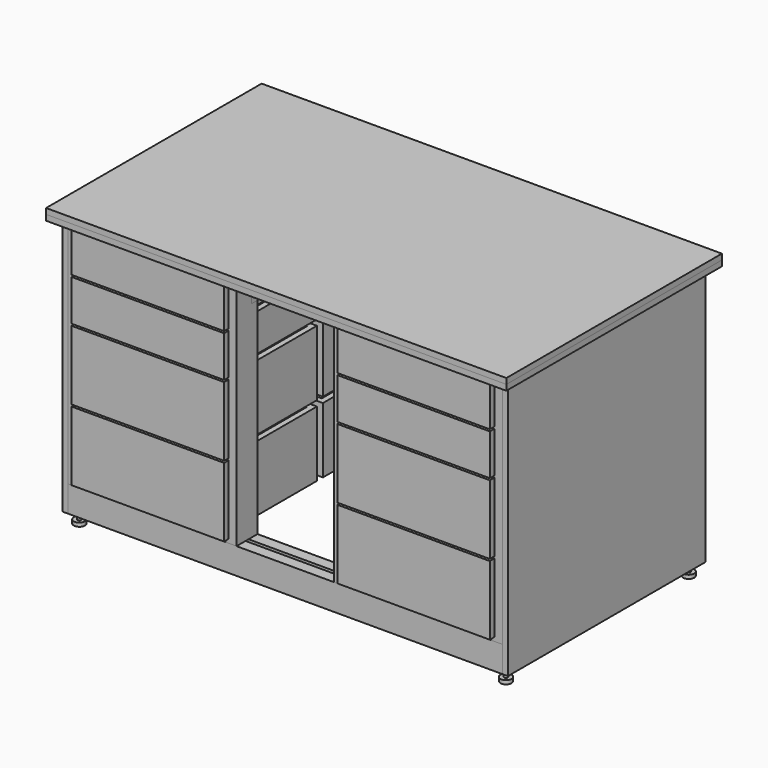
from build123d import *

# Parameters (mm, degrees)
F0_W      = 38.1
F0_H      = 88.9
F1_DEPTH  = 787.4
F2_W      = 38.1
F2_H      = 38.1
F2_W_2    = 1435.1
F3_DEPTH  = 88.9
F2_W_3    = 1473.2
F4_W      = 19.05
F4_H      = 838.2
F5_DEPTH  = 876.3
F6_W      = 38.1
F6_H      = 25.4
F7_DEPTH  = 88.9
F8_W      = 38.1
F8_H      = 685.8
F8_H_2    = 25.4
F9_DEPTH  = 88.9
F8_H_3    = 711.2
F11_DEPTH = 876.3
F12_DEPTH = 38.1
F10_W     = 1562.1
F10_H     = 19.05
F13_DEPTH = 876.3
F14_DEPTH = 38.1
F15_W     = 428.625
F15_H     = 127
F16_DEPTH = 19.05
F18_DEPTH = 127
F19_W     = 428.625
F19_H     = 368.3
F20_DEPTH = 9.525
F21_W     = 466.725
F21_H     = 127
F22_DEPTH = 19.05
F25_W     = 428.625
F25_H     = 222.25
F26_DEPTH = 19.05
F28_DEPTH = 222.25
F29_W     = 428.625
F29_H     = 368.3
F30_DEPTH = 19.05
F31_W     = 517.525
F31_H     = 234.95
F32_DEPTH = 19.05
F61_W     = 76.2
F61_H     = 12.7
F62_DEPTH = 88.9
F63_R     = 6.35
F64_DEPTH = 25.4
F65_R     = 19.05
F66_DEPTH = 12.7


# Not quite as in the source:
# - a feature names something its author has since deleted; it is built from what else it names


with BuildPart() as f1:
    # F0 (on Top) → F1 (new body)
    with BuildSketch(Plane.XY):
        with Locations((-717.55, 374.65)):
            Rectangle(F0_W, F0_H)
    extrude(amount=F1_DEPTH)


with BuildPart() as f1b:
    # F0 (on Top) → F1, piece 2 (new body)
    with BuildSketch(Plane.XY):
        with Locations((717.55, 374.65)):
            Rectangle(F0_W, F0_H)
    extrude(amount=F1_DEPTH)


with BuildPart() as f1c:
    # F0 (on Top) → F1, piece 3 (new body)
    with BuildSketch(Plane.XY):
        with Locations((717.55, -374.65)):
            Rectangle(F0_W, F0_H)
    extrude(amount=F1_DEPTH)


with BuildPart() as f1d:
    # F0 (on Top) → F1, piece 4 (new body)
    with BuildSketch(Plane.XY):
        with Locations((-717.55, -374.65)):
            Rectangle(F0_W, F0_H)
    extrude(amount=F1_DEPTH)


with BuildPart() as f1e:
    # F0 (on Top) → F1, piece 5 (new body)
    with BuildSketch(Plane.XY):
        with Locations((-184.15, 374.65)):
            Rectangle(F0_W, F0_H)
    extrude(amount=F1_DEPTH)


with BuildPart() as f1f:
    # F0 (on Top) → F1, piece 6 (new body)
    with BuildSketch(Plane.XY):
        with Locations((184.15, 374.65)):
            Rectangle(F0_W, F0_H)
    extrude(amount=F1_DEPTH)


with BuildPart() as f1g:
    # F0 (on Top) → F1, piece 7 (new body)
    with BuildSketch(Plane.XY):
        with Locations((184.15, -374.65)):
            Rectangle(F0_W, F0_H)
    extrude(amount=F1_DEPTH)


with BuildPart() as f1h:
    # F0 (on Top) → F1, piece 8 (new body)
    with BuildSketch(Plane.XY):
        with Locations((-184.15, -374.65)):
            Rectangle(F0_W, F0_H)
    extrude(amount=F1_DEPTH)


with BuildPart() as f3:
    # F2 (on face) → F3 (new body)
    with BuildSketch(Plane(origin=(0, 0, 0), x_dir=(1, 0, 0), z_dir=(0, 0, -1))):
        with Locations((-717.55, 349.25)):
            Rectangle(F2_W, F2_H)
        with Locations((19.05, 349.25)):
            Rectangle(F2_W_2, F2_H)
    extrude(amount=F3_DEPTH)


with BuildPart() as f3b:
    # F2 (on face) → F3, piece 2 (new body)
    with BuildSketch(Plane(origin=(0, 0, 0), x_dir=(1, 0, 0), z_dir=(0, 0, -1))):
        with Locations((19.05, 400.05)):
            Rectangle(F2_W_2, F2_H)
        with Locations((-717.55, 400.05)):
            Rectangle(F2_W, F2_H)
    extrude(amount=F3_DEPTH)


with BuildPart() as f3c:
    # F2 (on face) → F3, piece 3 (new body)
    with BuildSketch(Plane(origin=(0, 0, 0), x_dir=(1, 0, 0), z_dir=(0, 0, -1))):
        with Locations((0, -349.25)):
            Rectangle(F2_W_3, F2_H)
    extrude(amount=F3_DEPTH)


with BuildPart() as f3d:
    # F2 (on face) → F3, piece 4 (new body)
    with BuildSketch(Plane(origin=(0, 0, 0), x_dir=(1, 0, 0), z_dir=(0, 0, -1))):
        with Locations((0, -400.05)):
            Rectangle(F2_W_3, F2_H)
    extrude(amount=F3_DEPTH)


with BuildPart() as f5:
    # F4 (on face) → F5 (new body)
    with BuildSketch(Plane.XY.offset(787.4)):
        with Locations((746.125, 0)):
            Rectangle(F4_W, F4_H)
    extrude(amount=-F5_DEPTH)


with BuildPart() as f5b:
    # F4 (on face) → F5, piece 2 (new body)
    with BuildSketch(Plane.XY.offset(787.4)):
        Polygon((-736.6, 419.1), (-755.65, 419.1), (-755.65, -419.1), (-736.6, -419.1), (-736.6, 330.2), align=None)
    extrude(amount=-F5_DEPTH)


with BuildPart() as f7_tool:
    # F6 (on face) → F7 (new body)
    with BuildSketch(Plane.XY.offset(787.4)):
        with Locations((-717.55, 342.9)):
            Rectangle(F6_W, F6_H)
        with Locations((-184.15, 342.9)):
            Rectangle(F6_W, F6_H)
        with Locations((184.15, 342.9)):
            Rectangle(F6_W, F6_H)
        with Locations((717.55, 342.9)):
            Rectangle(F6_W, F6_H)
        with Locations((717.55, -342.9)):
            Rectangle(F6_W, F6_H)
        with Locations((184.15, -342.9)):
            Rectangle(F6_W, F6_H)
        with Locations((-184.15, -342.9)):
            Rectangle(F6_W, F6_H)
        with Locations((-717.55, -342.9)):
            Rectangle(F6_W, F6_H)
    extrude(amount=-F7_DEPTH)


with BuildPart() as f1_1:
    add(f1.part)

    # F7: cut by f7_tool
    add(f7_tool.part, mode=Mode.SUBTRACT)


with BuildPart() as f1b_1:
    add(f1b.part)

    # F7: cut by f7_tool
    add(f7_tool.part, mode=Mode.SUBTRACT)


with BuildPart() as f1c_1:
    add(f1c.part)

    # F7: cut by f7_tool
    add(f7_tool.part, mode=Mode.SUBTRACT)


with BuildPart() as f1d_1:
    add(f1d.part)

    # F7: cut by f7_tool
    add(f7_tool.part, mode=Mode.SUBTRACT)


with BuildPart() as f1e_1:
    add(f1e.part)

    # F7: cut by f7_tool
    add(f7_tool.part, mode=Mode.SUBTRACT)


with BuildPart() as f1f_1:
    add(f1f.part)

    # F7: cut by f7_tool
    add(f7_tool.part, mode=Mode.SUBTRACT)


with BuildPart() as f1g_1:
    add(f1g.part)

    # F7: cut by f7_tool
    add(f7_tool.part, mode=Mode.SUBTRACT)


with BuildPart() as f1h_1:
    add(f1h.part)

    # F7: cut by f7_tool
    add(f7_tool.part, mode=Mode.SUBTRACT)


with BuildPart() as f9:
    # F8 (on face) → F9 (new body)
    with BuildSketch(Plane.XY.offset(698.5)):
        with Locations((-717.55, -12.7)):
            Rectangle(F8_W, F8_H)
        with Locations((-717.55, 342.9)):
            Rectangle(F8_W, F8_H_2)
    extrude(amount=F9_DEPTH)


with BuildPart() as f9b:
    # F8 (on face) → F9, piece 2 (new body)
    with BuildSketch(Plane.XY.offset(698.5)):
        with Locations((-184.15, 0)):
            Rectangle(F8_W, F8_H_3)
    extrude(amount=F9_DEPTH)


with BuildPart() as f9c:
    # F8 (on face) → F9, piece 3 (new body)
    with BuildSketch(Plane.XY.offset(698.5)):
        with Locations((184.15, 0)):
            Rectangle(F8_W, F8_H_3)
    extrude(amount=F9_DEPTH)


with BuildPart() as f9d:
    # F8 (on face) → F9, piece 4 (new body)
    with BuildSketch(Plane.XY.offset(698.5)):
        with Locations((717.55, 0)):
            Rectangle(F8_W, F8_H_3)
    extrude(amount=F9_DEPTH)


with BuildPart() as f11:
    # F10 (on face) → F11 (new body)
    with BuildSketch(Plane.XZ.offset(419.1)):
        Polygon((781.05, 806.45), (-781.05, 806.45), (-781.05, 787.4), (-736.6, 787.4), (-698.5, 787.4), (781.05, 787.4), align=None)
    extrude(amount=-F11_DEPTH)

    # F10 (on face) → F12 (join)
    with BuildSketch(Plane.XZ.offset(419.1)):
        Polygon((781.05, 806.45), (-781.05, 806.45), (-781.05, 787.4), (-736.6, 787.4), (-698.5, 787.4), (781.05, 787.4), align=None)
    extrude(amount=F12_DEPTH)


with BuildPart() as f13:
    # F10 (on face) → F13 (new body)
    with BuildSketch(Plane.XZ.offset(419.1)):
        with Locations((0, 815.975)):
            Rectangle(F10_W, F10_H)
    extrude(amount=-F13_DEPTH)

    # F10 (on face) → F14 (join)
    with BuildSketch(Plane.XZ.offset(419.1)):
        with Locations((0, 815.975)):
            Rectangle(F10_W, F10_H)
    extrude(amount=F14_DEPTH)


with BuildPart() as f16:
    # F15 (on face) → F16 (new body)
    with BuildSketch(Plane.XZ.offset(419.1)):
        with Locations((-450.85, 704.85)):
            Rectangle(F15_W, F15_H)
    extrude(amount=-F16_DEPTH)

    # F17 (on face) → F18 (join)
    with BuildSketch(Plane.XY.offset(768.35)):
        Polygon((-665.1625, -400.05), (-665.1625, -31.75), (-684.2125, -31.75), (-684.2125, -419.1), (-665.1625, -419.1), align=None)
        Polygon((-217.4875, -31.75), (-236.5375, -31.75), (-236.5375, -400.05), (-236.5375, -419.1), (-217.4875, -419.1), align=None)
        Polygon((-665.1625, -31.75), (-236.5375, -31.75), (-217.4875, -31.75), (-217.4875, -12.7), (-684.2125, -12.7), (-684.2125, -31.75), align=None)
    extrude(amount=-F18_DEPTH)

    # F19 (on face) → F20 (join)
    with BuildSketch(Plane(origin=(0, 0, 641.35), x_dir=(1, 0, 0), z_dir=(0, 0, -1))):
        with Locations((-450.85, 215.9)):
            Rectangle(F19_W, F19_H)
    extrude(amount=-F20_DEPTH)


with BuildPart() as f22:
    # F21 (on face) → F22 (new body)
    with BuildSketch(Plane.XZ.offset(419.1)):
        with Locations((-450.85, 704.85)):
            Rectangle(F21_W, F21_H)
        Polygon((-192.0875, 781.05), (-709.6125, 781.05), (-709.6125, 641.35), (-684.2125, 641.35), (-684.2125, 768.35), (-217.4875, 768.35), (-217.4875, 641.35), (-192.0875, 641.35), align=None)
    extrude(amount=F22_DEPTH)


with BuildPart() as f23_1:
    # F23: copy of F16
    add(f16.part.moved(Location((0, 0, -146.05))))


with BuildPart() as f24_1:
    # F24: copy of F22
    add(f22.part.moved(Location((0, 0, -146.05))))


with BuildPart() as f26:
    # F25 (on face) → F26 (new body)
    with BuildSketch(Plane.XZ.offset(419.1)):
        with Locations((-450.85, 365.125)):
            Rectangle(F25_W, F25_H)
    extrude(amount=-F26_DEPTH)

    # F27 (on face) → F28 (join)
    with BuildSketch(Plane.XY.offset(476.25)):
        Polygon((-684.2125, -419.1), (-665.1625, -419.1), (-665.1625, -400.05), (-665.1625, -31.75), (-684.2125, -31.75), align=None)
        Polygon((-236.5375, -400.05), (-236.5375, -419.1), (-217.4875, -419.1), (-217.4875, -31.75), (-236.5375, -31.75), align=None)
        Polygon((-236.5375, -31.75), (-217.4875, -31.75), (-217.4875, -12.7), (-684.2125, -12.7), (-684.2125, -31.75), (-665.1625, -31.75), align=None)
    extrude(amount=-F28_DEPTH)

    # F29 (on face) → F30 (join)
    with BuildSketch(Plane(origin=(0, 0, 254), x_dir=(1, 0, 0), z_dir=(0, 0, -1))):
        with Locations((-450.85, 215.9)):
            Rectangle(F29_W, F29_H)
    extrude(amount=-F30_DEPTH)


with BuildPart() as f32:
    # F31 (on face) → F32 (new body)
    with BuildSketch(Plane.XZ.offset(419.1)):
        with Locations((-450.85, 371.475)):
            Rectangle(F31_W, F31_H)
    extrude(amount=F32_DEPTH)


with BuildPart() as f33_1:
    # F33: copy of F32
    add(f32.part.moved(Location((0, 0, -241.3))))


with BuildPart() as f34_1:
    # F34: copy of F26
    add(f26.part.moved(Location((0, 0, -241.3))))


with BuildPart() as f35_1:
    # F35: copy of F34_1
    add(f34_1.part.moved(Location((901.7, 0, 0))))


with BuildPart() as f36_1:
    # F36: copy of F33_1
    add(f33_1.part.moved(Location((901.7, 0, 0))))


with BuildPart() as f37_1:
    # F37: copy of F16
    add(f16.part.moved(Location((901.7, 0, 0))))


with BuildPart() as f38_1:
    # F38: copy of F22
    add(f22.part.moved(Location((901.7, 0, 0))))


with BuildPart() as f39_1:
    # F39: copy of F24_1
    add(f24_1.part.moved(Location((901.7, 0, 0))))


with BuildPart() as f40_1:
    # F40: copy of F23_1
    add(f23_1.part.moved(Location((901.7, 0, 0))))


with BuildPart() as f41_1:
    # F41: copy of F26
    add(f26.part.moved(Location((901.7, 0, 0))))


with BuildPart() as f42_1:
    # F42: copy of F32
    add(f32.part.moved(Location((901.7, 0, 0))))


with BuildPart() as f43_1:
    # F43: copy of F16
    add(f16.part.moved(Location((0, 412.75, 0))))


with BuildPart() as f45_1:
    # F45: copy of F16
    add(f16.part.moved(Location((0, 431.8, 0))))


with BuildPart() as f46_1:
    # F46: copy of F22
    add(f22.part.moved(Location((0, 857.25, 0))))


with BuildPart() as f47_1:
    # F47: copy of F23_1
    add(f23_1.part.moved(Location((0, 431.8, 0))))


with BuildPart() as f48_1:
    # F48: copy of F24_1
    add(f24_1.part.moved(Location((0, 857.25, 0))))


with BuildPart() as f49_1:
    # F49: copy of F26
    add(f26.part.moved(Location((0, 431.8, 0))))


with BuildPart() as f50_1:
    # F50: copy of F32
    add(f32.part.moved(Location((0, 857.25, 0))))


with BuildPart() as f51_1:
    # F51: copy of F34_1
    add(f34_1.part.moved(Location((0, 431.8, 0))))


with BuildPart() as f52_1:
    # F52: copy of F33_1
    add(f33_1.part.moved(Location((0, 857.25, 0))))


with BuildPart() as f53_1:
    # F53: copy of F37_1
    add(f37_1.part.moved(Location((0, 431.8, 0))))


with BuildPart() as f54_1:
    # F54: copy of F38_1
    add(f38_1.part.moved(Location((0, 857.25, 0))))


with BuildPart() as f55_1:
    # F55: copy of F40_1
    add(f40_1.part.moved(Location((0, 431.8, 0))))


with BuildPart() as f56_1:
    # F56: copy of F39_1
    add(f39_1.part.moved(Location((0, 857.25, 0))))


with BuildPart() as f57_1:
    # F57: copy of F41_1
    add(f41_1.part.moved(Location((0, 431.8, 0))))


with BuildPart() as f58_1:
    # F58: copy of F42_1
    add(f42_1.part.moved(Location((0, 857.25, 0))))


with BuildPart() as f59_1:
    # F59: copy of F35_1
    add(f35_1.part.moved(Location((0, 431.8, 0))))


with BuildPart() as f60_1:
    # F60: copy of F36_1
    add(f36_1.part.moved(Location((0, 857.25, 0))))


with BuildPart() as f62:
    # F61 (on face) → F62 (new body)
    with BuildSketch(Plane(origin=(0, 0, -88.9), x_dir=(1, 0, 0), z_dir=(0, 0, -1))):
        with Locations((-698.5, 374.65)):
            Rectangle(F61_W, F61_H)
    extrude(amount=-F62_DEPTH)


with BuildPart() as f62b:
    # F61 (on face) → F62, piece 2 (new body)
    with BuildSketch(Plane(origin=(0, 0, -88.9), x_dir=(1, 0, 0), z_dir=(0, 0, -1))):
        with Locations((698.5, 374.65)):
            Rectangle(F61_W, F61_H)
    extrude(amount=-F62_DEPTH)


with BuildPart() as f62c:
    # F61 (on face) → F62, piece 3 (new body)
    with BuildSketch(Plane(origin=(0, 0, -88.9), x_dir=(1, 0, 0), z_dir=(0, 0, -1))):
        with Locations((698.5, -374.65)):
            Rectangle(F61_W, F61_H)
    extrude(amount=-F62_DEPTH)


with BuildPart() as f62d:
    # F61 (on face) → F62, piece 4 (new body)
    with BuildSketch(Plane(origin=(0, 0, -88.9), x_dir=(1, 0, 0), z_dir=(0, 0, -1))):
        with Locations((-698.5, -374.65)):
            Rectangle(F61_W, F61_H)
    extrude(amount=-F62_DEPTH)


with BuildPart() as f64:
    # F63 (on face) → F64 (new body)
    with BuildSketch(Plane(origin=(0, 0, -88.9), x_dir=(1, 0, 0), z_dir=(0, 0, -1))):
        with Locations((-723.9, 387.35)):
            Circle(F63_R)
    extrude(amount=F64_DEPTH)


with BuildPart() as f64b:
    # F63 (on face) → F64, piece 2 (new body)
    with BuildSketch(Plane(origin=(0, 0, -88.9), x_dir=(1, 0, 0), z_dir=(0, 0, -1))):
        with Locations((723.9, 387.35)):
            Circle(F63_R)
    extrude(amount=F64_DEPTH)


with BuildPart() as f64c:
    # F63 (on face) → F64, piece 3 (new body)
    with BuildSketch(Plane(origin=(0, 0, -88.9), x_dir=(1, 0, 0), z_dir=(0, 0, -1))):
        with Locations((-723.9, -387.35)):
            Circle(F63_R)
    extrude(amount=F64_DEPTH)


with BuildPart() as f64d:
    # F63 (on face) → F64, piece 4 (new body)
    with BuildSketch(Plane(origin=(0, 0, -88.9), x_dir=(1, 0, 0), z_dir=(0, 0, -1))):
        with Locations((723.9, -387.35)):
            Circle(F63_R)
    extrude(amount=F64_DEPTH)


with BuildPart() as f66:
    # F65 (on face) → F66 (new body)
    with BuildSketch(Plane(origin=(0, 0, -114.3), x_dir=(1, 0, 0), z_dir=(0, 0, -1))):
        with Locations((-723.9, 387.35)):
            Circle(F65_R)
    extrude(amount=F66_DEPTH)


with BuildPart() as f66b:
    # F65 (on face) → F66, piece 2 (new body)
    with BuildSketch(Plane(origin=(0, 0, -114.3), x_dir=(1, 0, 0), z_dir=(0, 0, -1))):
        with Locations((723.9, 387.35)):
            Circle(F65_R)
    extrude(amount=F66_DEPTH)


with BuildPart() as f66c:
    # F65 (on face) → F66, piece 3 (new body)
    with BuildSketch(Plane(origin=(0, 0, -114.3), x_dir=(1, 0, 0), z_dir=(0, 0, -1))):
        with Locations((-723.9, -387.35)):
            Circle(F65_R)
    extrude(amount=F66_DEPTH)


with BuildPart() as f66d:
    # F65 (on face) → F66, piece 4 (new body)
    with BuildSketch(Plane(origin=(0, 0, -114.3), x_dir=(1, 0, 0), z_dir=(0, 0, -1))):
        with Locations((723.9, -387.35)):
            Circle(F65_R)
    extrude(amount=F66_DEPTH)


solid = Compound([f3.part, f3b.part, f3c.part, f3d.part, f5.part, f5b.part, f1_1.part, f1b_1.part, f1c_1.part, f1d_1.part, f1e_1.part, f1f_1.part, f1g_1.part, f1h_1.part, f9.part, f9b.part, f9c.part, f9d.part, f11.part, f13.part, f16.part, f22.part, f23_1.part, f24_1.part, f26.part, f32.part, f33_1.part, f34_1.part, f35_1.part, f36_1.part, f37_1.part, f38_1.part, f39_1.part, f40_1.part, f41_1.part, f42_1.part, f45_1.part, f46_1.part, f47_1.part, f48_1.part, f49_1.part, f50_1.part, f51_1.part, f52_1.part, f53_1.part, f54_1.part, f55_1.part, f56_1.part, f57_1.part, f58_1.part, f59_1.part, f60_1.part, f62.part, f62b.part, f62c.part, f62d.part, f64.part, f64b.part, f64c.part, f64d.part, f66.part, f66b.part, f66c.part, f66d.part])
